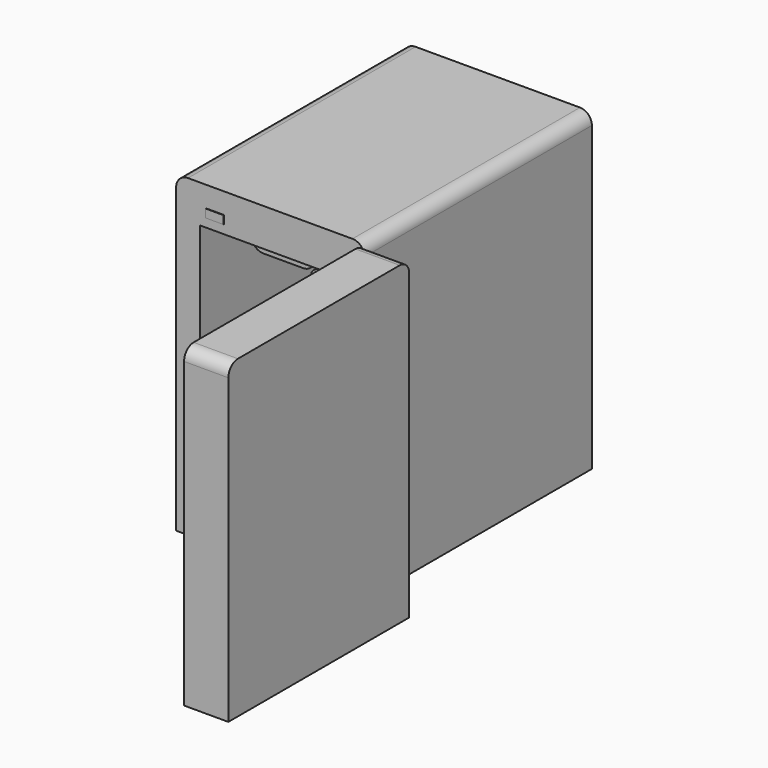
from build123d import *

# Parameters (mm, degrees)
F0_W         = 80.1943540573
F0_H         = 121.1211308837
F1_DEPTH     = 133.858
F2_W         = 18.8613273203
F2_H         = 96.3003262877
F3_DEPTH     = 134.112
F4_W         = 64.1634315252
F4_H         = 29.464147985
F4_W_2       = 63.6551976204
F4_H_2       = 34.9228568375
F5_DEPTH     = 13.97
F6_W         = 1.7585195601
F6_H         = 64.1634315252
F7_DEPTH     = 9.8044
F8_W         = 2.3097619414
F8_H         = 63.6551976204
F9_DEPTH     = 13.843
F10_R        = 5.08
F10_2_R      = 5.08
F11_W        = 7.8514143825
F11_H        = 7.4035450816
F11_H_2      = 8.0685932189
F12_DEPTH    = 7.62
F13_R        = 5.08
F14_W        = 64.35992755
F14_H        = 51.1236339808
F14_W_2      = 64.5319614559
F14_H_2      = 47.8723710403
F15_DEPTH    = 68.072
F16_DEPTH    = 7.112
F17_W        = 28.1689930707
F17_H        = 53.517022583
F17_W_2      = 36.3629683852
F18_DEPTH    = 12.7
F19_R        = 5.08
F20_W        = 7.7713597566
F20_H        = 3.5107582808
F21_DEPTH    = 0.2286
F22_W        = 26.9276434556
F22_H        = 11.6446465254
F23_DEPTH    = 4.2418
F24_T1_DEPTH = 36.6965031233
F25_R        = 3.6178439309
F26_DEPTH    = 18.9738
F27_W        = 5.2568218671
F27_H        = 8.7943524122
F28_DEPTH    = 11.2268


# Not quite as in the source:
# - a fillet or chamfer that OpenCascade refuses, or shapes differently, is made with other operations: its cross-section is extruded or revolved along the edge and cut away or added


with BuildPart() as f1:
    # F0 (on Top) → F1 (new body)
    with BuildSketch(Plane.XY):
        with Locations((1.6591921449, -10.5082280934)):
            Rectangle(F0_W, F0_H)
    extrude(amount=F1_DEPTH)

    # F10
    f10_edges = [f1.edges().sort_by_distance(p)[0] for p in [
        (-38.437985, -10.508228, 133.858),
        (41.756369, -10.508228, 133.858),
    ]]
    fillet(f10_edges, radius=F10_R)

    # F11 (on face) → F12 (join)
    with BuildSketch(Plane.YZ.offset(41.7563691735)):
        with Locations((-67.143086344, 107.1041934192)):
            Rectangle(F11_W, F11_H)
        with Locations((-67.143086344, 20.0026882812)):
            Rectangle(F11_W, F11_H_2)
    extrude(amount=F12_DEPTH)

    # F13
    f13_edges = [f1.edges().sort_by_distance(p)[0] for p in [
        (49.376369, -63.217379, 107.104193),
        (49.376369, -63.217379, 20.002688),
    ]]
    fillet(f13_edges, radius=F13_R)

    # F14 (on face) → F15 (cut)
    with BuildSketch(Plane.XZ.offset(71.0687935352)):
        with Locations((4.0109707043, 92.2216698527)):
            Rectangle(F14_W, F14_H)
        with Locations((4.0969876572, 34.6483555622)):
            Rectangle(F14_W_2, F14_H_2)
    extrude(amount=-F15_DEPTH, mode=Mode.SUBTRACT)

    # F16 (cut): a face of the model
    f16_faces = [f1.faces().sort_by_distance(p)[0] for p in [
        (4.0109707043, -37.0327935352, 66.6598528624),
    ]]
    extrude(f16_faces, amount=-F16_DEPTH, mode=Mode.SUBTRACT)

    # F17 (on face) → F18 (join)
    with BuildSketch(Plane.XY.offset(10.7121700421)):
        with Locations((-14.0844965354, -29.7553048267)):
            Rectangle(F17_W, F17_H)
        with Locations((18.1814841926, -29.7553048267)):
            Rectangle(F17_W_2, F17_H)
    extrude(amount=F18_DEPTH)

    # F19
    f19_edges = [f1.edges().sort_by_distance(p)[0] for p in [
        (4.096988, -56.513816, 23.41217),
    ]]
    fillet(f19_edges, radius=F19_R)

    # F20 (on face) → F21 (join)
    with BuildSketch(Plane.XZ.offset(71.0687935352)):
        with Locations((-21.8933494762, 123.2520565391)):
            Rectangle(F20_W, F20_H)
    extrude(amount=F21_DEPTH)

    # F22 (on face) → F23 (join)
    with BuildSketch(Plane(origin=(0, 0, 117.7834868431), x_dir=(1, 0, 0), z_dir=(0, 0, -1))):
        with Locations((4.1761337779, 61.5042597055)):
            Rectangle(F22_W, F22_H)
    extrude(amount=F23_DEPTH)

    # F24: fillet of radius 5.08 on 2 edges, made by hand

    # F24_s2 → F24_t1 (cut)
    with BuildSketch(Plane.XZ.offset(43.1560081439)):
        with BuildLine():
            ThreePointArc((-9.2876879498, 117.7834868431), (-7.559720018, 114.7445451124), (-4.2773166303, 113.5416868431))
            Line((-4.2773166303, 113.5416868431), (-9.2876879498, 113.5416868431))
            Line((-9.2876879498, 113.5416868431), (-9.2876879498, 117.7834868431))
        make_face()
        with BuildLine():
            ThreePointArc((17.6399555057, 117.7834868431), (15.9119875739, 114.7445451124), (12.6295841862, 113.5416868431))
            Line((12.6295841862, 113.5416868431), (17.6399555057, 113.5416868431))
            Line((17.6399555057, 113.5416868431), (17.6399555057, 117.7834868431))
        make_face()
    extrude(amount=F24_T1_DEPTH, mode=Mode.SUBTRACT)

    # F25 (on face) → F26 (join)
    with BuildSketch(Plane.XY.offset(59.5478528624)):
        with Locations((-22.0553409308, -13.7025229633)):
            Circle(F25_R)
    extrude(amount=F26_DEPTH)

    # F27 (on face) → F28 (join)
    with BuildSketch(Plane.XY.offset(59.5478528624)):
        with Locations((-5.8286509011, -13.5883204639)):
            Rectangle(F27_W, F27_H)
    extrude(amount=F28_DEPTH)


with BuildPart() as f3:
    # F2 (on Top) → F3 (new body)
    with BuildSketch(Plane.XY):
        with Locations((51.7478492111, -119.6234412491)):
            Rectangle(F2_W, F2_H)
    extrude(amount=F3_DEPTH)

    # F4 (on face) → F5 (cut)
    with BuildSketch(Plane(origin=(42.3171855509, 0, 0), x_dir=(0, -1, 0), z_dir=(-1, 0, 0))):
        with Locations((121.580503881, 100.977037102)):
            Rectangle(F4_W, F4_H)
        with Locations((121.8346208334, 39.7402029485)):
            Rectangle(F4_W_2, F4_H_2)
    extrude(amount=-F5_DEPTH, mode=Mode.SUBTRACT)

    # F6 (on face) → F7 (join)
    with BuildSketch(Plane.XY.offset(86.2449631095)):
        with Locations((43.196445331, -121.580503881)):
            Rectangle(F6_W, F6_H)
    extrude(amount=F7_DEPTH)

    # F8 (on face) → F9 (join)
    with BuildSketch(Plane.XY.offset(22.2787745297)):
        with Locations((43.4720665216, -121.8346208334)):
            Rectangle(F8_W, F8_H)
    extrude(amount=F9_DEPTH)

    # F10#2
    f10_2_edges = [f3.edges().sort_by_distance(p)[0] for p in [
        (51.747849, -167.773604, 134.112),
        (51.747849, -71.473278, 134.112),
    ]]
    fillet(f10_2_edges, radius=F10_2_R)


solid = Compound([f1.part, f3.part])
